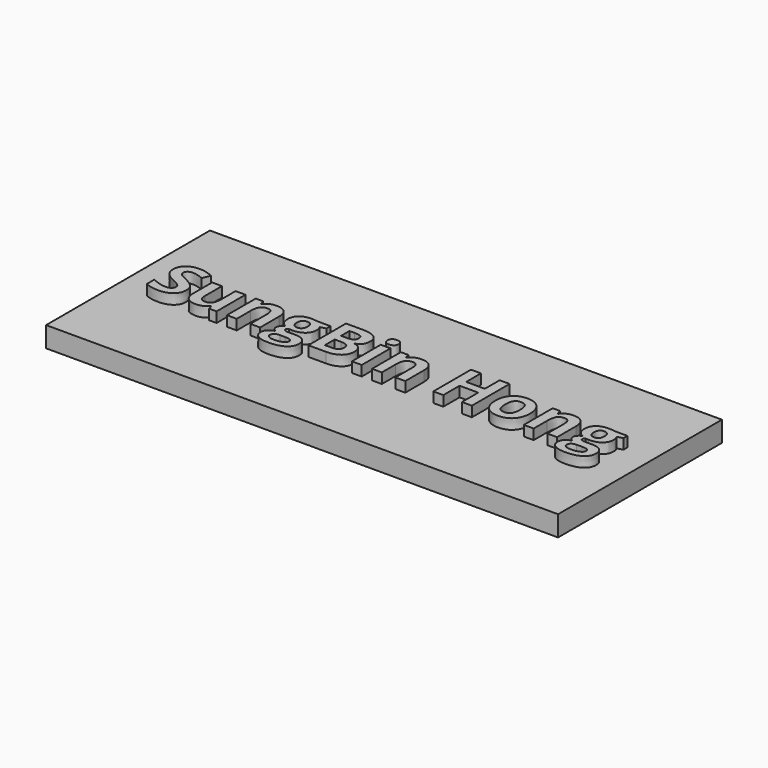
from build123d import *

# Parameters (mm, degrees)
F0_W         = 50
F0_H         = 20
F1_DEPTH     = 2
F2_TEXT_SIZE = 6.4433854621
F3_DEPTH     = 1


# Not quite as in the source:
# - Text() gives the source's letters only with a copy of the font that has no kerning and outlines rounded to 1/6400 em; it was checked with that copy


with BuildPart() as f1:
    # F0 (on Top) → F1 (new body)
    with BuildSketch(Plane.XY):
        with Locations((25, 10)):
            Rectangle(F0_W, F0_H)
    extrude(amount=F1_DEPTH)

    # F2 (on face) → F3 (join)
    with BuildSketch(Plane.XY.offset(2)):
        with Locations((2.6589367419, 8.3919876136)):
            Text('SungBin Hong', F2_TEXT_SIZE, font='Open Sans', font_style=FontStyle.BOLD, text_align=(TextAlign.LEFT, TextAlign.BOTTOM))
    extrude(amount=F3_DEPTH)


solid = f1.part
